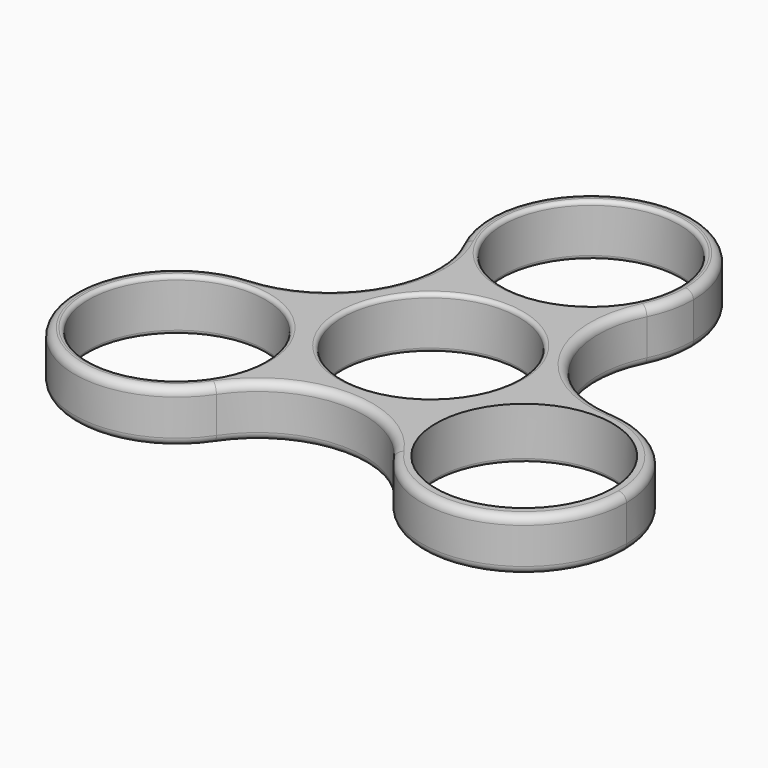
from build123d import *

# Parameters (mm, degrees)
F0_R     = 11
F1_DEPTH = 6.5
F2_R     = 1
F3_R     = 0.5


with BuildPart() as f1:
    # F0 (on Top) → F1 (new body)
    with BuildSketch(Plane.XY):
        with BuildLine():
            ThreePointArc((12.0815519999, -4.0741381018), (12.5817782527, -2.0643052101), (12.75, 0))
            ThreePointArc((12.75, 0), (9.8639869866, 8.0786298794), (2.5124689053, 12.5))
            ThreePointArc((2.5124689053, 12.5), (0, 12.25), (-2.5124689053, 12.5))
            ThreePointArc((-2.5124689053, 12.5), (-11.0418238983, 6.375), (-12.0815519999, -4.0741381018))
            ThreePointArc((-12.0815519999, -4.0741381018), (-10.6088111964, -6.125), (-9.5690830947, -8.4258618982))
            ThreePointArc((-9.5690830947, -8.4258618982), (0, -12.75), (9.5690830947, -8.4258618982))
            ThreePointArc((9.5690830947, -8.4258618982), (10.6088111964, -6.125), (12.0815519999, -4.0741381018))
        make_face()
        Circle(F0_R, mode=Mode.SUBTRACT)
        with BuildLine():
            ThreePointArc((2.5124689053, 12.5), (9.8639869866, 8.0786298794), (12.75, 0))
            ThreePointArc((12.75, 0), (12.5817782527, -2.0643052101), (12.0815519999, -4.0741381018))
            ThreePointArc((12.0815519999, -4.0741381018), (16.7895332065, -0.7130500793), (22.4981276547, 0.2218024022))
            ThreePointArc((22.4981276547, 0.2218024022), (11.8579416889, 6.8461856384), (11.4411501987, 19.3730485936))
            ThreePointArc((11.4411501987, 19.3730485936), (7.7772469915, 14.896687215), (2.5124689053, 12.5))
        make_face()
        with BuildLine():
            ThreePointArc((-2.5124689053, 12.5), (0, 12.25), (2.5124689053, 12.5))
            ThreePointArc((2.5124689053, 12.5), (0, 12.75), (-2.5124689053, 12.5))
        make_face()
        with BuildLine():
            ThreePointArc((-2.5124689053, 12.5), (0, 12.75), (2.5124689053, 12.5))
            ThreePointArc((2.5124689053, 12.5), (7.7772469915, 14.896687215), (11.4411501987, 19.3730485936))
            ThreePointArc((11.4411501987, 19.3730485936), (12.4184774637, 22.1114160073), (12.75, 25))
            ThreePointArc((12.75, 25), (-2.8885839653, 37.4184774701), (-11.4411502236, 19.3730486441))
            ThreePointArc((-11.4411502236, 19.3730486441), (-7.7772470139, 14.8966872321), (-2.5124689053, 12.5))
        make_face()
        with Locations((0, 25)):
            Circle(F0_R, mode=Mode.SUBTRACT)
        with BuildLine():
            ThreePointArc((22.4981276547, 0.2218024022), (16.7895332065, -0.7130500793), (12.0815519999, -4.0741381018))
            ThreePointArc((12.0815519999, -4.0741381018), (11.0418238983, -6.375), (9.5690830947, -8.4258618982))
            ThreePointArc((9.5690830947, -8.4258618982), (9.0122859979, -14.1836365732), (11.0569765695, -19.5948501784))
            ThreePointArc((11.0569765695, -19.5948501784), (25.3582862247, -24.6990091031), (34.4006350946, -12.5))
            ThreePointArc((34.4006350946, -12.5), (30.9610601692, -3.7891742682), (22.4981276547, 0.2218024022))
        make_face()
        with Locations((21.6506350946, -12.5)):
            Circle(F0_R, mode=Mode.SUBTRACT)
        with BuildLine():
            ThreePointArc((9.5690830947, -8.4258618982), (11.0418238983, -6.375), (12.0815519999, -4.0741381018))
            ThreePointArc((12.0815519999, -4.0741381018), (10.6088111964, -6.125), (9.5690830947, -8.4258618982))
        make_face()
        with BuildLine():
            ThreePointArc((-12.0815519999, -4.0741381018), (-11.0418238983, 6.375), (-2.5124689053, 12.5))
            ThreePointArc((-2.5124689053, 12.5), (-7.7772470139, 14.8966872321), (-11.4411502236, 19.3730486441))
            ThreePointArc((-11.4411502236, 19.3730486441), (-10.4210792392, 16.514917487), (-10.0750574606, 13.5))
            ThreePointArc((-10.0750574606, 13.5), (-13.6650642316, 4.4082012887), (-22.498128058, 0.2218023753))
            ThreePointArc((-22.498128058, 0.2218023753), (-16.7895333933, -0.7130500022), (-12.0815519999, -4.0741381018))
        make_face()
        with BuildLine():
            ThreePointArc((11.0569765695, -19.5948501784), (9.0122859979, -14.1836365732), (9.5690830947, -8.4258618982))
            ThreePointArc((9.5690830947, -8.4258618982), (0, -12.75), (-9.5690830947, -8.4258618982))
            ThreePointArc((-9.5690830947, -8.4258618982), (-9.0688568419, -10.4356947899), (-8.9006350946, -12.5))
            ThreePointArc((-8.9006350946, -12.5), (-9.4516260346, -16.207651272), (-11.0569767345, -19.5948504248))
            ThreePointArc((-11.0569767345, -19.5948504248), (-1.483e-07, -13.6923715584), (11.0569765695, -19.5948501784))
        make_face()
        with BuildLine():
            ThreePointArc((-9.5690830947, -8.4258618982), (-10.6088111964, -6.125), (-12.0815519999, -4.0741381018))
            ThreePointArc((-12.0815519999, -4.0741381018), (-11.0418238983, -6.375), (-9.5690830947, -8.4258618982))
        make_face()
        with BuildLine():
            ThreePointArc((-9.5690830947, -8.4258618982), (-11.0418238983, -6.375), (-12.0815519999, -4.0741381018))
            ThreePointArc((-12.0815519999, -4.0741381018), (-16.7895333933, -0.7130500022), (-22.498128058, 0.2218023753))
            ThreePointArc((-22.498128058, 0.2218023753), (-32.6924586322, -18.8750006247), (-11.0569767345, -19.5948504248))
            ThreePointArc((-11.0569767345, -19.5948504248), (-9.4516260346, -16.207651272), (-8.9006350946, -12.5))
            ThreePointArc((-8.9006350946, -12.5), (-9.0688568419, -10.4356947899), (-9.5690830947, -8.4258618982))
        make_face()
        with Locations((-21.6506350946, -12.5)):
            Circle(F0_R, mode=Mode.SUBTRACT)
    extrude(amount=F1_DEPTH)

    # F2
    f2_edges = [f1.edges().sort_by_distance(p)[0] for p in [
        (0, 37.75, 6.5),
        (0, 37.75, 0),
        (32.692459, -18.875001, 0),
        (32.692459, -18.875001, 6.5),
        (11.857942, 6.846186, 0),
        (11.857942, 6.846186, 6.5),
        (-11.857942, 6.846185, 0),
        (-11.857942, 6.846185, 6.5),
        (-32.692459, -18.875001, 0),
        (-32.692459, -18.875001, 6.5),
        (0, -13.692372, 0),
        (0, -13.692372, 6.5),
    ]]
    fillet(f2_edges, radius=F2_R)

    # F3
    f3_edges = [f1.edges().sort_by_distance(p)[0] for p in [
        (-11, 25, 6.5),
        (-11, 0, 6.5),
        (-32.650635, -12.5, 6.5),
        (-11, 25, 0),
        (-11, 0, 0),
        (-32.650635, -12.5, 0),
        (10.650635, -12.5, 0),
    ]]
    fillet(f3_edges, radius=F3_R)


solid = f1.part
